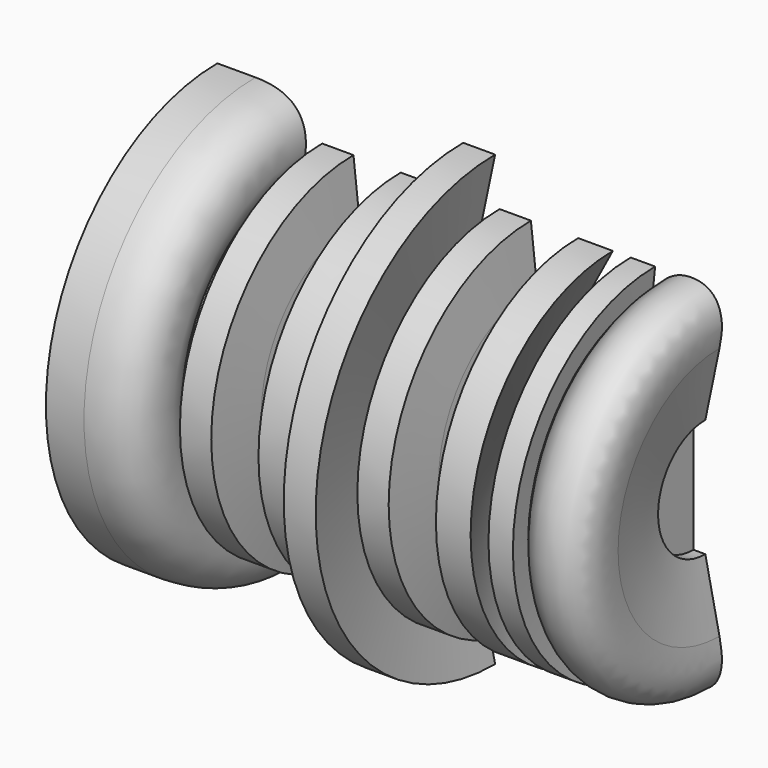
from build123d import *

# Parameters (mm, degrees)
F0_TEXT_SIZE = 64.7532921802
F1_ANGLE     = 180
F3_ANGLE     = 180


# Not quite as in the source:
# - Text() gives the source's letters only with a copy of the font that has no kerning and outlines rounded to 1/6400 em; it was checked with that copy


with BuildPart() as f1:
    # F0 (on Front) → F1 (revolve)
    with BuildSketch(Plane.XZ):
        with Locations((-73.8438181579, 17.596184276)):
            Text('Rylyn', F0_TEXT_SIZE, font='Open Sans', font_style=FontStyle.BOLDITALIC, text_align=(TextAlign.LEFT, TextAlign.BOTTOM))
    revolve(axis=Axis((1.0527633131, 0, 0), (1, 0, 0)), revolution_arc=F1_ANGLE)

    # F2 (on Front) → F3 (revolve)
    with BuildSketch(Plane.XZ):
        Polygon((-67.7143782377, 0), (79.3716683984, 0), (79.3716683984, 19.4009207189), (55.6093044579, 19.4009207189), (30.9445671737, 3.759868443), (22.5224606693, 3.759868443), (16.2058826536, 7.0685525425), (9.5885135233, 19.4009207189), (2.6703542098, 19.4009207189), (-22.0784256106, 6.469021138), (-35.8306989074, 3.1582894735), (-39.740961045, 19.4009207189), (-67.7143782377, 19.4009207189), align=None)
    revolve(axis=Axis((5.8286450803, 0, 0), (1, 0, 0)), revolution_arc=F3_ANGLE)


solid = f1.part
